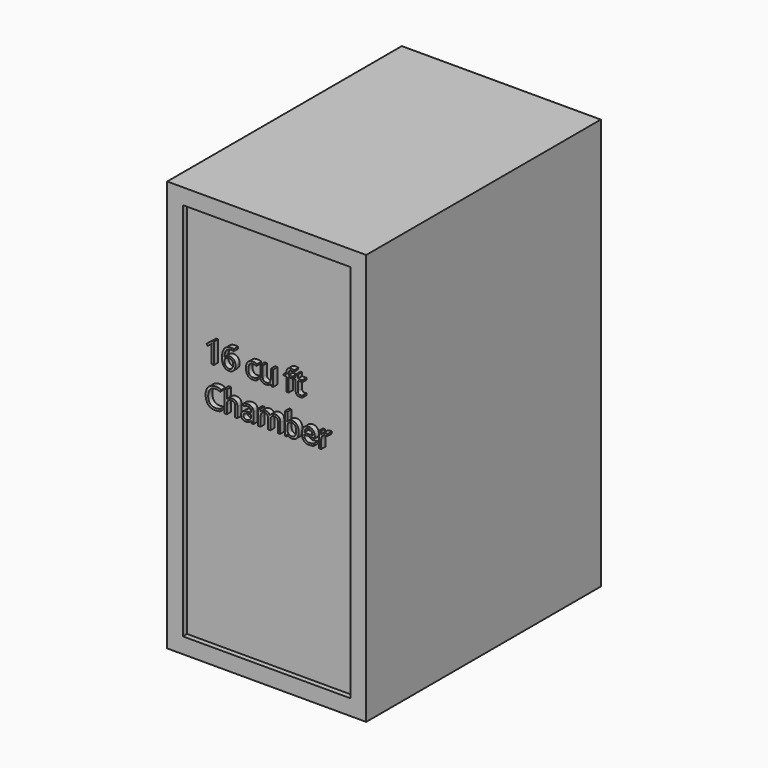
from build123d import *

# Parameters (mm, degrees)
F0_W         = 965.2
F0_H         = 1422.4
F1_DEPTH     = 1993.9
F2_W         = 812.8
F2_H         = 1841.5
F3_DEPTH     = 25.4
F4_TEXT_SIZE = 139.6963620739
F5_DEPTH     = 25.4


# Not quite as in the source:
# - Text() gives the source's letters only with a copy of the font that has no kerning and outlines rounded to 1/6400 em; it was checked with that copy


with BuildPart() as f1:
    # F0 (on Top) → F1 (new body)
    with BuildSketch(Plane.XY):
        Rectangle(F0_W, F0_H)
    extrude(amount=F1_DEPTH)

    # F2 (on face) → F3 (cut)
    with BuildSketch(Plane.XZ.offset(711.2)):
        with Locations((0, 996.95)):
            Rectangle(F2_W, F2_H)
    extrude(amount=-F3_DEPTH, mode=Mode.SUBTRACT)

    # F4 (on face) → F5 (join)
    with BuildSketch(Plane.XZ.offset(685.8)):
        with Locations((-304.8, 1283.7186193068)):
            Text('16 cu ft', F4_TEXT_SIZE, font='Open Sans', text_align=(TextAlign.LEFT, TextAlign.BOTTOM))
        with Locations((-304.8, 1093.7315668863)):
            Text('Chamber', F4_TEXT_SIZE, font='Open Sans', text_align=(TextAlign.LEFT, TextAlign.BOTTOM))
    extrude(amount=F5_DEPTH)


solid = f1.part
